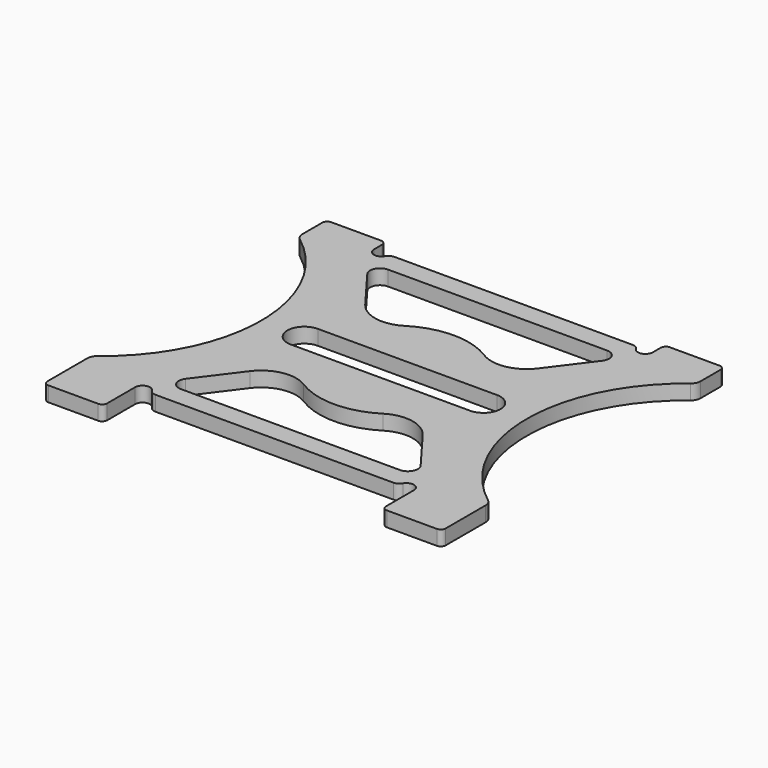
from build123d import *

# Parameters (mm, degrees)
F1_DEPTH = 1.5


# Not quite as in the source:
# - ends of sketch curves that miss each other by under 0.0002 mm in the source are joined


with BuildPart() as f1:
    # F0 (on Top) → F1 (new body)
    with BuildSketch(Plane.XY):
        with BuildLine():
            ThreePointArc((19.6082164698, -11.4503983868), (13.339608, 1.2499996959), (19.608215987, 13.9503980169))
            ThreePointArc((19.608215987, 13.9503980169), (19.8967236619, 14.3015730303), (20.000004, 14.744172))
            Line((20.000004, 14.744172), (20.000004, 17.25))
            ThreePointArc((20.000004, 17.25), (19.8535573906, 17.6035533906), (19.500004, 17.75))
            Line((19.500004, 17.75), (14.500004, 17.75))
            ThreePointArc((14.500004, 17.75), (14.1464506094, 17.6035533906), (14.000004, 17.25))
            Line((14.000004, 17.25), (14.000004, 16.25))
            ThreePointArc((14.000004, 16.25), (13.4441182966, 15.5255556337), (12.6004849604, 15.8749999771))
            ThreePointArc((12.6004849604, 15.8749999771), (12.3259659886, 16.1495190594), (11.950966, 16.25))
            Line((11.950966, 16.25), (-11.950958, 16.25))
            ThreePointArc((-11.950958, 16.25), (-12.3259579886, 16.1495190594), (-12.6004770396, 15.8750000229))
            ThreePointArc((-12.6004770396, 15.8750000229), (-13.4441102966, 15.5255556337), (-13.999996, 16.25))
            Line((-13.999996, 16.25), (-13.999996, 17.25))
            ThreePointArc((-13.999996, 17.25), (-14.1464426094, 17.6035533906), (-14.499996, 17.75))
            Line((-14.499996, 17.75), (-19.499996, 17.75))
            ThreePointArc((-19.499996, 17.75), (-19.8535493906, 17.6035533906), (-19.999996, 17.25))
            Line((-19.999996, 17.25), (-19.999996, 14.744172))
            ThreePointArc((-19.999996, 14.744172), (-19.8967156619, 14.3015730303), (-19.6082083041, 13.9503976031))
            ThreePointArc((-19.6082083041, 13.9503976031), (-13.3396, 1.2499996959), (-19.6082084698, -11.4503983868))
            ThreePointArc((-19.6082084698, -11.4503983868), (-19.8967227718, -11.8015703601), (-20.000004, -12.244173))
            Line((-20.000004, -12.244173), (-19.999996, -17.25))
            ThreePointArc((-19.999996, -17.25), (-19.8535493906, -17.6035533906), (-19.499996, -17.75))
            Line((-19.499996, -17.75), (-14.499996, -17.75))
            ThreePointArc((-14.499996, -17.75), (-14.1464426094, -17.6035533906), (-13.999996, -17.25))
            Line((-13.999996, -17.25), (-13.999996, -13.75))
            ThreePointArc((-13.999996, -13.75), (-13.4441102966, -13.0255556337), (-12.6004769604, -13.3749999771))
            ThreePointArc((-12.6004769604, -13.3749999771), (-12.3259579886, -13.6495190594), (-11.950958, -13.75))
            Line((-11.950958, -13.75), (11.950966, -13.75))
            ThreePointArc((11.950966, -13.75), (12.3259659886, -13.6495190594), (12.6004850396, -13.3750000229))
            ThreePointArc((12.6004850396, -13.3750000229), (13.4441182966, -13.0255556337), (14.000004, -13.75))
            Line((14.000004, -13.75), (14.000004, -17.25))
            ThreePointArc((14.000004, -17.25), (14.1464506094, -17.6035533906), (14.500004, -17.75))
            Line((14.500004, -17.75), (19.500004, -17.75))
            ThreePointArc((19.500004, -17.75), (19.8535573906, -17.6035533906), (20.000004, -17.25))
            Line((20.000004, -17.25), (20.000004, -12.244173))
            ThreePointArc((20.000004, -12.244173), (19.8967236619, -11.8015740303), (19.6082164698, -11.4503983868))
        make_face()
        with BuildLine():
            ThreePointArc((-8.6748168, -5.9830934), (-6.4973578405, -4.6318753463), (-3.9800720916, -5.1118651461))
            ThreePointArc((-3.9800720916, -5.1118651461), (3.5765e-06, -6.257042), (3.980079547, -5.1118658719))
            ThreePointArc((3.980079547, -5.1118658719), (6.4973651354, -4.631875401), (8.67482416, -5.98309388))
            Line((8.67482416, -5.98309388), (11.800004, -10.15))
            ThreePointArc((11.800004, -10.15), (11.894431191, -11.1972135955), (11.000004, -11.75))
            Line((11.000004, -11.75), (-10.999996, -11.75))
            ThreePointArc((-10.999996, -11.75), (-11.894423191, -11.1972135955), (-11.799996, -10.15))
            Line((-11.799996, -10.15), (-8.6748168, -5.9830934))
        make_face(mode=Mode.SUBTRACT)
        with BuildLine():
            ThreePointArc((9.000004, 2.95), (10.700004, 1.25), (9.000004, -0.45))
            Line((9.000004, -0.45), (-8.999996, -0.45))
            ThreePointArc((-8.999996, -0.45), (-10.699996, 1.25), (-8.999996, 2.95))
            Line((-8.999996, 2.95), (9.000004, 2.95))
        make_face(mode=Mode.SUBTRACT)
        with BuildLine():
            Line((-10.999996, 14.25), (11.000004, 14.25))
            ThreePointArc((11.000004, 14.25), (11.894431191, 13.6972135955), (11.800004, 12.65))
            Line((11.800004, 12.65), (8.674824, 8.483093))
            ThreePointArc((8.674824, 8.483093), (6.4973648742, 7.1318743525), (3.9800786415, 7.6118644285))
            ThreePointArc((3.9800786415, 7.6118644285), (3.5765e-06, 8.757041), (-3.9800718144, 7.6118647041))
            ThreePointArc((-3.9800718144, 7.6118647041), (-6.4973575792, 7.1318742978), (-8.6748168, 8.4830924))
            Line((-8.6748168, 8.4830924), (-11.799996, 12.65))
            ThreePointArc((-11.799996, 12.65), (-11.894423191, 13.6972135955), (-10.999996, 14.25))
        make_face(mode=Mode.SUBTRACT)
    extrude(amount=F1_DEPTH)


solid = f1.part
